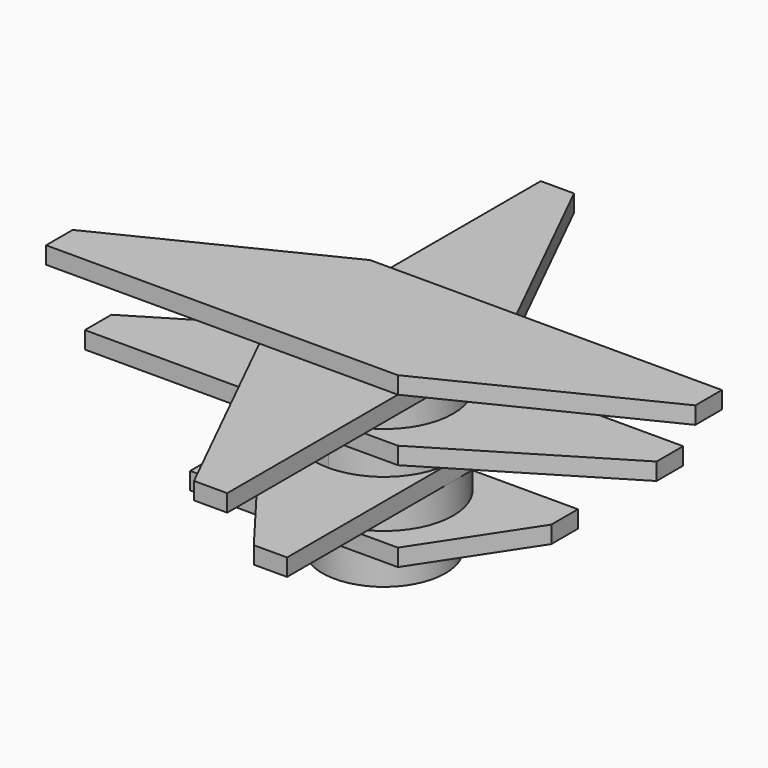
from build123d import *

# Parameters (mm, degrees)
F1_DEPTH  = 6.2
F3_DEPTH  = 6.2
F5_DEPTH  = 10
F7_DEPTH  = 6.2
F9_DEPTH  = 9
F11_DEPTH = 6.2
F13_DEPTH = 11
F15_DEPTH = 6.2
F16_R     = 22.25
F17_DEPTH = 13
F19_D     = 35
F19_DEPTH = 35
F19_TIP   = 10.515060833


# Not quite as in the source:
# - a feature names something its author has since deleted; it is built from what else it names


with BuildPart() as f1:
    # F0 (on Top) → F1 (new body)
    with BuildSketch(Plane.XY):
        Polygon((11.0905365064, -25), (25, -25), (102, 13), (102, 25), (11.0905365064, 25), (-11.0905365064, 25), (-25, 25), (-102, -13), (-102, -25), (-11.0905365064, -25), align=None)
    extrude(amount=F1_DEPTH)

    # F2 (on face) → F3 (join)
    with BuildSketch(Plane(origin=(0, 0, 0), x_dir=(1, 0, 0), z_dir=(0, 0, -1))):
        Polygon((-25, 25), (-25, 0), (-25, -25), (25, -25), (25, 0), (25, 25), align=None)
        Polygon((25, -25), (-25, -25), (-25, -102), (-13, -102), align=None)
        Polygon((13, 102), (-25, 25), (25, 25), (25, 102), align=None)
    extrude(amount=F3_DEPTH)

    # F4 (on face) → F5 (join)
    with BuildSketch(Plane(origin=(0, 0, -6.2), x_dir=(1, 0, 0), z_dir=(0, 0, -1))):
        with BuildLine():
            ThreePointArc((-25, 2.61e-08), (-1.3e-08, -25), (25, 0))
            ThreePointArc((25, 0), (1.3e-08, 25), (-25, 2.61e-08))
        make_face()
    extrude(amount=F5_DEPTH)

    # F6 (on face) → F7 (join)
    with BuildSketch(Plane(origin=(0, 0, -16.2), x_dir=(1, 0, 0), z_dir=(0, 0, -1))):
        with BuildLine():
            Line((-5.83e-08, -25), (25, -25))
            Line((25, -25), (25, 0))
            ThreePointArc((25, 0), (17.677669509, -17.6776695503), (-5.83e-08, -25))
        make_face()
        with BuildLine():
            Line((-25, -25), (-5.83e-08, -25))
            ThreePointArc((-5.83e-08, -25), (-17.6776695503, -17.677669509), (-25, 0))
            Line((-25, 0), (-25, -25))
        make_face()
        Polygon((25, 0), (25, -25), (88, -25), (88, -13), (25, 25), align=None)
        Polygon((-88, 13), (-25, -25), (-25, 0), (-25, 25), (-88, 25), align=None)
        with BuildLine():
            ThreePointArc((-25, 0), (-17.6776695503, -17.677669509), (-5.83e-08, -25))
            ThreePointArc((-5.83e-08, -25), (17.677669509, -17.6776695503), (25, 0))
            ThreePointArc((25, 0), (17.6776695297, 17.6776695297), (0, 25))
            ThreePointArc((0, 25), (-17.6776695297, 17.6776695297), (-25, 0))
        make_face()
        with BuildLine():
            Line((-25, 25), (-25, 0))
            ThreePointArc((-25, 0), (-17.6776695297, 17.6776695297), (0, 25))
            Line((0, 25), (-25, 25))
        make_face()
        with BuildLine():
            ThreePointArc((0, 25), (17.6776695297, 17.6776695297), (25, 0))
            Line((25, 0), (25, 25))
            Line((25, 25), (0, 25))
        make_face()
    extrude(amount=F7_DEPTH)

    # F8 (on face) → F9 (join)
    with BuildSketch(Plane(origin=(0, 0, -22.4), x_dir=(1, 0, 0), z_dir=(0, 0, -1))):
        with BuildLine():
            ThreePointArc((-5.83e-08, -25), (17.677669509, -17.6776695503), (25, 0))
            ThreePointArc((25, 0), (17.6776695297, 17.6776695297), (0, 25))
            ThreePointArc((0, 25), (-25, 2.92e-08), (-5.83e-08, -25))
        make_face()
    extrude(amount=F9_DEPTH)

    # F10 (on face) → F11 (join)
    with BuildSketch(Plane(origin=(0, 0, -31.4), x_dir=(1, 0, 0), z_dir=(0, 0, -1))):
        Polygon((13, 75), (-25, 25), (4.22e-08, 25), (25, 25), (25, 75), align=None)
        with BuildLine():
            ThreePointArc((4.22e-08, 25), (17.6776695446, 17.6776695147), (25, 0))
            Line((25, 0), (25, 25))
            Line((25, 25), (4.22e-08, 25))
        make_face()
        with BuildLine():
            ThreePointArc((-25, 0), (-17.6776695332, -17.6776695262), (-9.9e-09, -25))
            ThreePointArc((-9.9e-09, -25), (17.6776695262, -17.6776695332), (25, 0))
            ThreePointArc((25, 0), (17.6776695446, 17.6776695147), (4.22e-08, 25))
            ThreePointArc((4.22e-08, 25), (-17.6776695147, 17.6776695446), (-25, 0))
        make_face()
        with BuildLine():
            ThreePointArc((25, 0), (17.6776695262, -17.6776695332), (-9.9e-09, -25))
            Line((-9.9e-09, -25), (25, -25))
            Line((25, -25), (25, 0))
        make_face()
        Polygon((-9.9e-09, -25), (-25, -25), (-25, -75), (-13, -75), (25, -25), align=None)
        with BuildLine():
            Line((-25, 0), (-25, -25))
            Line((-25, -25), (-9.9e-09, -25))
            ThreePointArc((-9.9e-09, -25), (-17.6776695332, -17.6776695262), (-25, 0))
        make_face()
        with BuildLine():
            Line((-25, 25), (-25, 0))
            ThreePointArc((-25, 0), (-17.6776695147, 17.6776695446), (4.22e-08, 25))
            Line((4.22e-08, 25), (-25, 25))
        make_face()
    extrude(amount=F11_DEPTH)

    # F12 (on face) → F13 (join)
    with BuildSketch(Plane(origin=(0, 0, -37.6), x_dir=(1, 0, 0), z_dir=(0, 0, -1))):
        with BuildLine():
            ThreePointArc((-25, 2.61e-08), (-1.3e-08, -25), (25, 0))
            ThreePointArc((25, 0), (1.3e-08, 25), (-25, 2.61e-08))
        make_face()
    extrude(amount=F13_DEPTH)

    # F14 (on face) → F15 (join)
    with BuildSketch(Plane(origin=(0, 0, -48.6), x_dir=(1, 0, 0), z_dir=(0, 0, -1))):
        with BuildLine():
            ThreePointArc((-25, 0), (-17.6776695204, -17.6776695389), (2.61e-08, -25))
            ThreePointArc((2.61e-08, -25), (17.6776695389, -17.6776695204), (25, 0))
            ThreePointArc((25, 0), (17.6776695389, 17.6776695204), (2.61e-08, 25))
            ThreePointArc((2.61e-08, 25), (-17.6776695204, 17.6776695389), (-25, 0))
        make_face()
        with BuildLine():
            ThreePointArc((2.61e-08, 25), (17.6776695389, 17.6776695204), (25, 0))
            Line((25, 0), (25, 25))
            Line((25, 25), (2.61e-08, 25))
        make_face()
        with BuildLine():
            Line((2.61e-08, -25), (25, -25))
            Line((25, -25), (25, 0))
            ThreePointArc((25, 0), (17.6776695389, -17.6776695204), (2.61e-08, -25))
        make_face()
        with BuildLine():
            Line((-25, -25), (2.61e-08, -25))
            ThreePointArc((2.61e-08, -25), (-17.6776695204, -17.6776695389), (-25, 0))
            Line((-25, 0), (-25, -25))
        make_face()
        with BuildLine():
            Line((-25, 25), (-25, 0))
            ThreePointArc((-25, 0), (-17.6776695204, 17.6776695389), (2.61e-08, 25))
            Line((2.61e-08, 25), (-25, 25))
        make_face()
        Polygon((-50, 13), (-25, -25), (-25, 0), (-25, 25), (-50, 25), align=None)
        Polygon((25, 0), (25, -25), (50, -25), (50, -13), (25, 25), align=None)
    extrude(amount=F15_DEPTH)

    # F16 (on face) → F17 (join)
    with BuildSketch(Plane(origin=(0, 0, -54.8), x_dir=(1, 0, 0), z_dir=(0, 0, -1))):
        Circle(F16_R)
    extrude(amount=F17_DEPTH)

    # F19
    with Locations(Plane(origin=(0, 0, -67.8), x_dir=(1, 0, 0), z_dir=(0, 0, -1))):
        with Locations((0, 0)):
            Hole(F19_D / 2, depth=F19_DEPTH)
            with Locations((0, 0, -(F19_DEPTH + F19_TIP / 2))):  # 118° drill point
                Cone(0, F19_D / 2, F19_TIP, mode=Mode.SUBTRACT)


solid = f1.part
